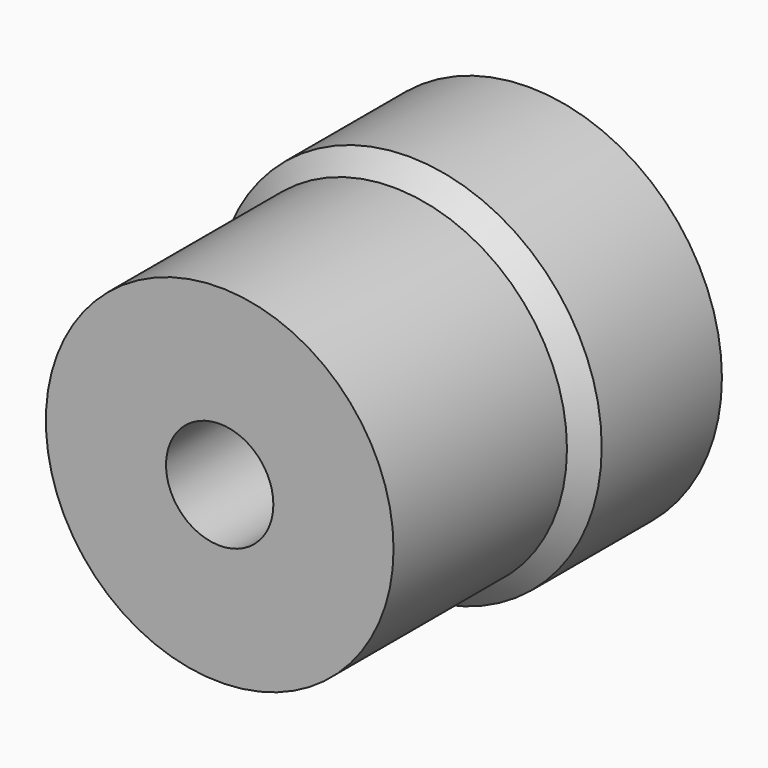
from build123d import *

# Parameters (mm, degrees)
F0_R        = 9
F1_DEPTH    = 8
F2_R        = 8.1
F3_DEPTH    = 10
F4_S5_R     = 8.1
F4_T6_DEPTH = 14
F5_R        = 2.5
F6_DEPTH    = 18.001


# Not quite as in the source:
# - a fillet or chamfer that OpenCascade refuses, or shapes differently, is made with other operations: its cross-section is extruded or revolved along the edge and cut away or added


with BuildPart() as f1:
    # F0 (on Front) → F1 (new body)
    with BuildSketch(Plane.XZ):
        Circle(F0_R)
    extrude(amount=F1_DEPTH)

    # F2 (on face) → F3 (join)
    with BuildSketch(Plane.XZ.offset(8)):
        Circle(F2_R)
    extrude(amount=F3_DEPTH)

    # F4: chamfer of 1 on 1 edges, made by hand


with BuildPart() as f4_tool2:
    # F4_s3 → F4_t4 (revolve)
    with BuildSketch(Plane.XY):
        Polygon((9, -7), (8, -8), (9, -8), align=None)
    revolve(axis=Axis((0, -8, 0), (0, -1, 0)))

    # F4_s5 → F4_t6 (cut, symmetric)
    with BuildSketch(Plane.XZ.offset(7.5)):
        Circle(F4_S5_R)
    extrude(amount=F4_T6_DEPTH, both=True, mode=Mode.SUBTRACT)


with BuildPart() as f1_1:
    add(f1.part)

    # F4_t1: cut F4_tool2
    add(f4_tool2.part, mode=Mode.SUBTRACT)

    # F5 (on face) → F6 (cut, through all)
    with BuildSketch(Plane.XZ.offset(18)):
        Circle(F5_R)
    extrude(amount=-F6_DEPTH, mode=Mode.SUBTRACT)


solid = f1_1.part
